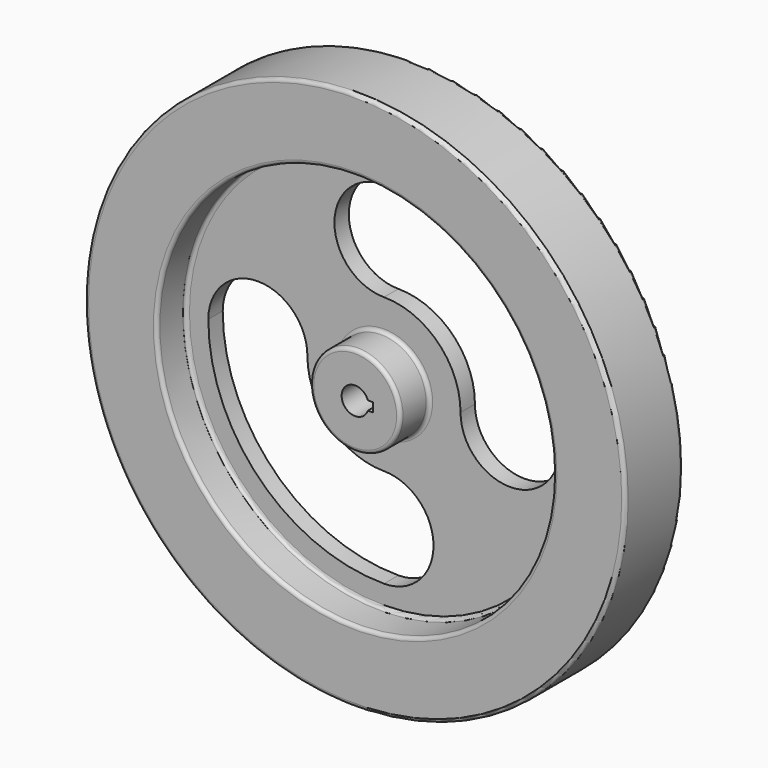
from build123d import *

# Parameters (mm, degrees)
F0_R     = 381
F1_DEPTH = 12.7
F2_R     = 381
F2_R_2   = 279.4
F2_R_3   = 63.5
F3_DEPTH = 50.8
F6_DEPTH = 25.4
F7_R     = 5.08
F9_DEPTH = 101.6


# Not quite as in the source:
# - a feature names something its author has since deleted; it is built from what else it names


with BuildPart() as f1:
    # F0 (on Front) → F1 (new body, symmetric)
    with BuildSketch(Plane.XZ):
        Circle(F0_R)
    extrude(amount=F1_DEPTH, both=True)

    # F2 (on face) → F3 (join, symmetric)
    with BuildSketch(Plane.XZ.offset(12.7)):
        Circle(F2_R)
        Circle(F2_R_2, mode=Mode.SUBTRACT)
        Circle(F2_R_3)
    extrude(amount=F3_DEPTH, both=True)

    # F5 (on face) → F6 (cut)
    with BuildSketch(Plane.XZ.offset(12.7)):
        with BuildLine():
            ThreePointArc((107.95, 0), (177.8, 69.85), (247.65, 0))
            ThreePointArc((247.65, 0), (175.1149943608, 175.1149943608), (0, 247.65))
            ThreePointArc((0, 247.65), (49.3914086659, 227.1914086659), (69.85, 177.8))
            ThreePointArc((69.85, 177.8), (49.3914086659, 128.4085913342), (2e-10, 107.95))
            ThreePointArc((2e-10, 107.95), (76.3321770291, 76.332177029), (107.95, 0))
        make_face()
        with BuildLine():
            ThreePointArc((-247.65, -7.01e-08), (-175.1149941454, -175.1149945763), (5.392e-07, -247.65))
            ThreePointArc((5.392e-07, -247.65), (-69.85, -177.7999999633), (6.127e-07, -107.95))
            ThreePointArc((6.127e-07, -107.95), (-76.3321768125, -76.3321772457), (-107.95, 0))
            ThreePointArc((-107.95, 0), (-177.799999965, -69.85), (-247.65, -7.01e-08))
        make_face()
        with BuildLine():
            ThreePointArc((69.85, 177.8), (49.3914086659, 227.1914086659), (0, 247.65))
            ThreePointArc((0, 247.65), (-69.85, 177.7999999999), (2e-10, 107.95))
            ThreePointArc((2e-10, 107.95), (49.3914086659, 128.4085913342), (69.85, 177.8))
        make_face()
        with BuildLine():
            ThreePointArc((-107.95, 0), (-177.800000035, 69.85), (-247.65, -7.01e-08))
            ThreePointArc((-247.65, -7.01e-08), (-177.799999965, -69.85), (-107.95, 0))
        make_face()
        with BuildLine():
            ThreePointArc((6.127e-07, -107.95), (-69.85, -177.7999999633), (5.392e-07, -247.65))
            ThreePointArc((5.392e-07, -247.65), (49.3914088565, -227.1914084752), (69.85, -177.8))
            ThreePointArc((69.85, -177.8), (49.3914088825, -128.4085915507), (6.127e-07, -107.95))
        make_face()
        with BuildLine():
            ThreePointArc((107.95, 0), (177.8, -69.85), (247.65, 0))
            ThreePointArc((247.65, 0), (177.8, 69.85), (107.95, 0))
        make_face()
    extrude(amount=-F6_DEPTH, mode=Mode.SUBTRACT)

    # F7
    f7_edges = [f1.edges().sort_by_distance(p)[0] for p in [
        (-63.5, -12.7, 0),
        (-279.4, -63.5, 0),
        (-381, -63.5, 0),
        (-63.5, 38.1, 0),
        (-381, 38.1, 0),
        (-279.4, 38.1, 0),
        (-279.4, -12.7, 0),
        (-63.5, -63.5, 0),
    ]]
    fillet(f7_edges, radius=F7_R)

    # F8 (on face) → F9 (cut)
    with BuildSketch(Plane.XZ.offset(63.5)):
        with BuildLine():
            ThreePointArc((17.9605122421, -6.35), (18.7756525614, -3.2213926947), (19.05, 0))
            ThreePointArc((19.05, 0), (18.7756525614, 3.2213926947), (17.9605122421, 6.35))
            Line((17.9605122421, 6.35), (-6.5611318409, 6.35))
            Line((-6.5611318409, 6.35), (-6.5611318409, -6.35))
            Line((-6.5611318409, -6.35), (17.9605122421, -6.35))
        make_face()
        with BuildLine():
            ThreePointArc((17.9605122421, 6.35), (18.7756525614, 3.2213926947), (19.05, 0))
            ThreePointArc((19.05, 0), (18.7756525614, -3.2213926947), (17.9605122421, -6.35))
            Line((17.9605122421, -6.35), (25.4, -6.35))
            Line((25.4, -6.35), (25.4, 6.35))
            Line((25.4, 6.35), (17.9605122421, 6.35))
        make_face()
        with BuildLine():
            Line((-6.5611318409, 6.35), (17.9605122421, 6.35))
            ThreePointArc((17.9605122421, 6.35), (-19.05, 0), (17.9605122421, -6.35))
            Line((17.9605122421, -6.35), (-6.5611318409, -6.35))
            Line((-6.5611318409, -6.35), (-6.5611318409, 6.35))
        make_face()
    extrude(amount=-F9_DEPTH, mode=Mode.SUBTRACT)


solid = f1.part
